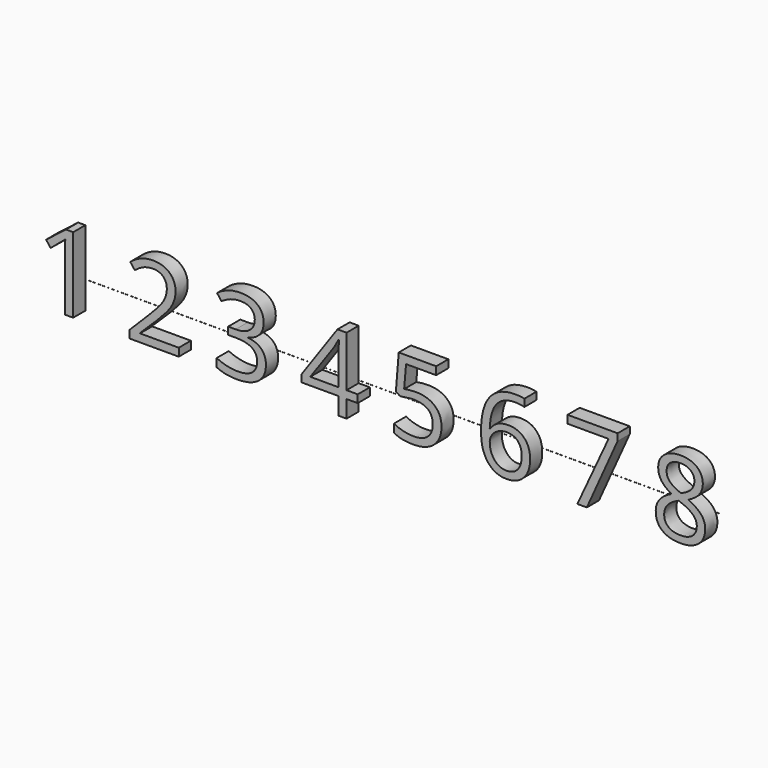
from build123d import *

# Parameters (mm, degrees)
F0_TEXT_SIZE = 20.8333333333
F1_DEPTH     = 3
F2_W         = 130
F2_H         = 0.01
F3_DEPTH     = 0.01


# Not quite as in the source:
# - Text() gives the source's letters only with a copy of the font that has no kerning and outlines rounded to 1/6400 em; it was checked with that copy


with BuildPart() as f1:
    # F0 (on Front) → F1 (new body)
    with BuildSketch(Plane.XZ):
        with Locations((0, 0)):
            Text('1 2 3 4 5 6 7 8', F0_TEXT_SIZE, font='Open Sans', text_align=(TextAlign.LEFT, TextAlign.BOTTOM))
    extrude(amount=F1_DEPTH)

    # F2 (on Front) → F3 (join)
    with BuildSketch(Plane.XZ):
        with Locations((68, 5.4655013712)):
            Rectangle(F2_W, F2_H)
    extrude(amount=F3_DEPTH)


solid = f1.part
